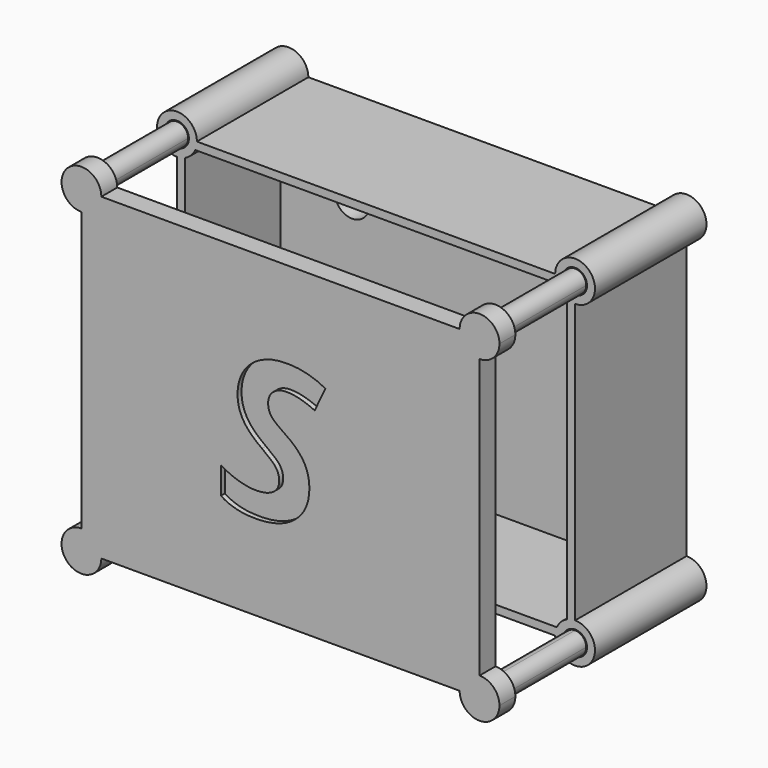
from build123d import *

# Parameters (mm, degrees)
F0_R         = 2.778125
F1_DEPTH     = 3.175
F2_DEPTH     = 22.225
F3_W         = 3.175
F3_H         = 50.8
F4_DEPTH     = 31.75
F6_DEPTH     = 3.175
F7_DEPTH     = 19.05
F5_TEXT_SIZE = 31.9108936108
F8_DEPTH     = 0.79375


# Not quite as in the source:
# - a length typed as a fraction of an inch, garbled in the dataset ("3 / 203.2 mm" for 3/8 in), is restored
# - Text() gives the source's letters only with a copy of the font that has no kerning and outlines rounded to 1/6400 em; it was checked with that copy


with BuildPart() as f1:
    # F0 (on Front) → F1 (new body)
    with BuildSketch(Plane.XZ):
        with BuildLine():
            Line((28.8400644337, 24.13), (-28.8400644337, 24.13))
            ThreePointArc((-28.8400644337, 24.13), (-29.5049359697, 23.1549359697), (-30.48, 22.4900644337))
            Line((-30.48, 22.4900644337), (-30.48, -22.4900644337))
            ThreePointArc((-30.48, -22.4900644337), (-29.5049359697, -23.1549359697), (-28.8400644337, -24.13))
            Line((-28.8400644337, -24.13), (28.8400644337, -24.13))
            ThreePointArc((28.8400644337, -24.13), (29.5049359697, -23.1549359697), (30.48, -22.4900644337))
            Line((30.48, -22.4900644337), (30.48, 22.4900644337))
            ThreePointArc((30.48, 22.4900644337), (29.5049359697, 23.1549359697), (28.8400644337, 24.13))
        make_face()
        with Locations((-19.05, 12.7)):
            Circle(F0_R, mode=Mode.SUBTRACT)
        with BuildLine():
            ThreePointArc((-30.48, 22.4900644337), (-31.1013168813, 22.2919724564), (-31.75, 22.225))
            Line((-31.75, 22.225), (-31.75, -22.225))
            ThreePointArc((-31.75, -22.225), (-31.1013168813, -22.2919724564), (-30.48, -22.4900644337))
            Line((-30.48, -22.4900644337), (-30.48, 22.4900644337))
        make_face()
        with BuildLine():
            ThreePointArc((-28.8400644337, 24.13), (-28.6419724564, 24.7513168813), (-28.575, 25.4))
            Line((-28.575, 25.4), (-29.845, 25.4))
            ThreePointArc((-29.845, 25.4), (-29.9704016562, 24.720253919), (-30.3300968343, 24.13))
            Line((-30.3300968343, 24.13), (-28.8400644337, 24.13))
        make_face()
        with BuildLine():
            Line((-29.845, 25.4), (-28.575, 25.4))
            ThreePointArc((-28.575, 25.4), (-33.9950640303, 27.6450640303), (-31.75, 22.225))
            Line((-31.75, 22.225), (-31.75, 23.495))
            ThreePointArc((-31.75, 23.495), (-33.0970384182, 26.7470384182), (-29.845, 25.4))
        make_face()
        with BuildLine():
            Line((28.575, 25.4), (-28.575, 25.4))
            ThreePointArc((-28.575, 25.4), (-28.6419724564, 24.7513168813), (-28.8400644337, 24.13))
            Line((-28.8400644337, 24.13), (28.8400644337, 24.13))
            ThreePointArc((28.8400644337, 24.13), (28.6419724564, 24.7513168813), (28.575, 25.4))
        make_face()
        with BuildLine():
            ThreePointArc((34.925, 25.4), (31.75, 28.575), (28.575, 25.4))
            Line((28.575, 25.4), (29.845, 25.4))
            ThreePointArc((29.845, 25.4), (31.75, 27.305), (33.655, 25.4))
            ThreePointArc((33.655, 25.4), (33.0970384182, 24.0529615818), (31.75, 23.495))
            Line((31.75, 23.495), (31.75, 22.225))
            ThreePointArc((31.75, 22.225), (33.9950640303, 23.1549359697), (34.925, 25.4))
        make_face()
        with BuildLine():
            Line((29.845, 25.4), (28.575, 25.4))
            ThreePointArc((28.575, 25.4), (28.6419724564, 24.7513168813), (28.8400644337, 24.13))
            Line((28.8400644337, 24.13), (30.3300968343, 24.13))
            ThreePointArc((30.3300968343, 24.13), (29.9704016562, 24.720253919), (29.845, 25.4))
        make_face()
        with BuildLine():
            Line((-31.75, 23.495), (-31.75, 22.225))
            ThreePointArc((-31.75, 22.225), (-31.1013168813, 22.2919724564), (-30.48, 22.4900644337))
            Line((-30.48, 22.4900644337), (-30.48, 23.9800968343))
            ThreePointArc((-30.48, 23.9800968343), (-31.070253919, 23.6204016562), (-31.75, 23.495))
        make_face()
        with BuildLine():
            ThreePointArc((-30.48, -22.4900644337), (-31.1013168813, -22.2919724564), (-31.75, -22.225))
            Line((-31.75, -22.225), (-31.75, -23.4950015545))
            ThreePointArc((-31.75, -23.4950015545), (-31.0702538242, -23.6204033564), (-30.48, -23.9800989199))
            Line((-30.48, -23.9800989199), (-30.48, -22.4900644337))
        make_face()
        with BuildLine():
            Line((-31.75, -23.4950015545), (-31.75, -22.225))
            ThreePointArc((-31.75, -22.225), (-33.9950640303, -27.6450640303), (-28.575, -25.4))
            Line((-28.575, -25.4), (-29.8450015545, -25.4))
            ThreePointArc((-29.8450015545, -25.4), (-33.097037319, -26.747037319), (-31.75, -23.4950015545))
        make_face()
        with BuildLine():
            ThreePointArc((30.48, 22.4900644337), (31.1013168813, 22.2919724564), (31.75, 22.225))
            Line((31.75, 22.225), (31.75, 23.495))
            ThreePointArc((31.75, 23.495), (31.070253919, 23.6204016562), (30.48, 23.9800968343))
            Line((30.48, 23.9800968343), (30.48, 22.4900644337))
        make_face()
        with BuildLine():
            Line((31.75, -22.225), (31.75, 22.225))
            ThreePointArc((31.75, 22.225), (31.1013168813, 22.2919724564), (30.48, 22.4900644337))
            Line((30.48, 22.4900644337), (30.48, -22.4900644337))
            ThreePointArc((30.48, -22.4900644337), (31.1013168813, -22.2919724564), (31.75, -22.225))
        make_face()
        with BuildLine():
            ThreePointArc((-28.8400644337, -24.13), (-28.6419724564, -24.7513168813), (-28.575, -25.4))
            Line((-28.575, -25.4), (28.575, -25.4))
            ThreePointArc((28.575, -25.4), (28.6419724564, -24.7513168813), (28.8400644337, -24.13))
            Line((28.8400644337, -24.13), (-28.8400644337, -24.13))
        make_face()
        with BuildLine():
            Line((-29.8450015545, -25.4), (-28.575, -25.4))
            ThreePointArc((-28.575, -25.4), (-28.6419724564, -24.7513168813), (-28.8400644337, -24.13))
            Line((-28.8400644337, -24.13), (-30.3300989199, -24.13))
            ThreePointArc((-30.3300989199, -24.13), (-29.9704033564, -24.7202538242), (-29.8450015545, -25.4))
        make_face()
        with BuildLine():
            ThreePointArc((34.925, -25.4), (33.9950640303, -23.1549359697), (31.75, -22.225))
            Line((31.75, -22.225), (31.75, -23.495))
            ThreePointArc((31.75, -23.495), (33.0970384182, -24.0529615818), (33.655, -25.4))
            ThreePointArc((33.655, -25.4), (31.75, -27.305), (29.845, -25.4))
            Line((29.845, -25.4), (28.575, -25.4))
            ThreePointArc((28.575, -25.4), (31.75, -28.575), (34.925, -25.4))
        make_face()
        with BuildLine():
            Line((31.75, -23.495), (31.75, -22.225))
            ThreePointArc((31.75, -22.225), (31.1013168813, -22.2919724564), (30.48, -22.4900644337))
            Line((30.48, -22.4900644337), (30.48, -23.9800968343))
            ThreePointArc((30.48, -23.9800968343), (31.070253919, -23.6204016562), (31.75, -23.495))
        make_face()
        with BuildLine():
            ThreePointArc((28.8400644337, -24.13), (28.6419724564, -24.7513168813), (28.575, -25.4))
            Line((28.575, -25.4), (29.845, -25.4))
            ThreePointArc((29.845, -25.4), (29.9704016562, -24.720253919), (30.3300968343, -24.13))
            Line((30.3300968343, -24.13), (28.8400644337, -24.13))
        make_face()
        with BuildLine():
            ThreePointArc((-30.48, 22.4900644337), (-29.5049359697, 23.1549359697), (-28.8400644337, 24.13))
            Line((-28.8400644337, 24.13), (-30.3300968343, 24.13))
            ThreePointArc((-30.3300968343, 24.13), (-30.4029615818, 24.0529615818), (-30.48, 23.9800968343))
            Line((-30.48, 23.9800968343), (-30.48, 22.4900644337))
        make_face()
        with BuildLine():
            ThreePointArc((-28.8400644337, -24.13), (-29.5049359697, -23.1549359697), (-30.48, -22.4900644337))
            Line((-30.48, -22.4900644337), (-30.48, -23.9800989199))
            ThreePointArc((-30.48, -23.9800989199), (-30.402962681, -24.052962681), (-30.3300989199, -24.13))
            Line((-30.3300989199, -24.13), (-28.8400644337, -24.13))
        make_face()
        with BuildLine():
            Line((30.48, -23.9800968343), (30.48, -22.4900644337))
            ThreePointArc((30.48, -22.4900644337), (29.5049359697, -23.1549359697), (28.8400644337, -24.13))
            Line((28.8400644337, -24.13), (30.3300968343, -24.13))
            ThreePointArc((30.3300968343, -24.13), (30.4029615818, -24.0529615818), (30.48, -23.9800968343))
        make_face()
        with BuildLine():
            Line((30.3300968343, 24.13), (28.8400644337, 24.13))
            ThreePointArc((28.8400644337, 24.13), (29.5049359697, 23.1549359697), (30.48, 22.4900644337))
            Line((30.48, 22.4900644337), (30.48, 23.9800968343))
            ThreePointArc((30.48, 23.9800968343), (30.4029615818, 24.0529615818), (30.3300968343, 24.13))
        make_face()
        with BuildLine():
            ThreePointArc((-30.3300968343, 24.13), (-29.9704016562, 24.720253919), (-29.845, 25.4))
            Line((-29.845, 25.4), (-31.75, 25.4))
            Line((-31.75, 25.4), (-31.75, 23.495))
            ThreePointArc((-31.75, 23.495), (-31.070253919, 23.6204016562), (-30.48, 23.9800968343))
            Line((-30.48, 23.9800968343), (-30.48, 24.13))
            Line((-30.48, 24.13), (-30.3300968343, 24.13))
        make_face()
        with BuildLine():
            Line((-31.75, 25.4), (-29.845, 25.4))
            ThreePointArc((-29.845, 25.4), (-33.0970384182, 26.7470384182), (-31.75, 23.495))
            Line((-31.75, 23.495), (-31.75, 25.4))
        make_face()
        with BuildLine():
            ThreePointArc((33.655, 25.4), (31.75, 27.305), (29.845, 25.4))
            Line((29.845, 25.4), (31.75, 25.4))
            Line((31.75, 25.4), (31.75, 23.495))
            ThreePointArc((31.75, 23.495), (33.0970384182, 24.0529615818), (33.655, 25.4))
        make_face()
        with BuildLine():
            Line((31.75, 25.4), (29.845, 25.4))
            ThreePointArc((29.845, 25.4), (29.9704016562, 24.720253919), (30.3300968343, 24.13))
            Line((30.3300968343, 24.13), (30.48, 24.13))
            Line((30.48, 24.13), (30.48, 23.9800968343))
            ThreePointArc((30.48, 23.9800968343), (31.070253919, 23.6204016562), (31.75, 23.495))
            Line((31.75, 23.495), (31.75, 25.4))
        make_face()
        with BuildLine():
            ThreePointArc((33.655, -25.4), (33.0970384182, -24.0529615818), (31.75, -23.495))
            Line((31.75, -23.495), (31.75, -25.4))
            Line((31.75, -25.4), (29.845, -25.4))
            ThreePointArc((29.845, -25.4), (31.75, -27.305), (33.655, -25.4))
        make_face()
        with BuildLine():
            Line((31.75, -25.4), (31.75, -23.495))
            ThreePointArc((31.75, -23.495), (31.070253919, -23.6204016562), (30.48, -23.9800968343))
            Line((30.48, -23.9800968343), (30.48, -24.13))
            Line((30.48, -24.13), (30.3300968343, -24.13))
            ThreePointArc((30.3300968343, -24.13), (29.9704016562, -24.720253919), (29.845, -25.4))
            Line((29.845, -25.4), (31.75, -25.4))
        make_face()
        with BuildLine():
            ThreePointArc((-30.48, -23.9800989199), (-31.0702538242, -23.6204033564), (-31.75, -23.4950015545))
            Line((-31.75, -23.4950015545), (-31.75, -25.4))
            Line((-31.75, -25.4), (-29.8450015545, -25.4))
            ThreePointArc((-29.8450015545, -25.4), (-29.9704033564, -24.7202538242), (-30.3300989199, -24.13))
            Line((-30.3300989199, -24.13), (-30.48, -24.13))
            Line((-30.48, -24.13), (-30.48, -23.9800989199))
        make_face()
        with BuildLine():
            Line((-31.75, -25.4), (-31.75, -23.4950015545))
            ThreePointArc((-31.75, -23.4950015545), (-33.097037319, -26.747037319), (-29.8450015545, -25.4))
            Line((-29.8450015545, -25.4), (-31.75, -25.4))
        make_face()
    extrude(amount=F1_DEPTH)

    # F0 (on Front) → F2 (join)
    with BuildSketch(Plane.XZ):
        with BuildLine():
            ThreePointArc((-30.48, 22.4900644337), (-31.1013168813, 22.2919724564), (-31.75, 22.225))
            Line((-31.75, 22.225), (-31.75, -22.225))
            ThreePointArc((-31.75, -22.225), (-31.1013168813, -22.2919724564), (-30.48, -22.4900644337))
            Line((-30.48, -22.4900644337), (-30.48, 22.4900644337))
        make_face()
        with BuildLine():
            ThreePointArc((-28.8400644337, -24.13), (-28.6419724564, -24.7513168813), (-28.575, -25.4))
            Line((-28.575, -25.4), (28.575, -25.4))
            ThreePointArc((28.575, -25.4), (28.6419724564, -24.7513168813), (28.8400644337, -24.13))
            Line((28.8400644337, -24.13), (-28.8400644337, -24.13))
        make_face()
        with BuildLine():
            Line((31.75, -22.225), (31.75, 22.225))
            ThreePointArc((31.75, 22.225), (31.1013168813, 22.2919724564), (30.48, 22.4900644337))
            Line((30.48, 22.4900644337), (30.48, -22.4900644337))
            ThreePointArc((30.48, -22.4900644337), (31.1013168813, -22.2919724564), (31.75, -22.225))
        make_face()
        with BuildLine():
            Line((28.575, 25.4), (-28.575, 25.4))
            ThreePointArc((-28.575, 25.4), (-28.6419724564, 24.7513168813), (-28.8400644337, 24.13))
            Line((-28.8400644337, 24.13), (28.8400644337, 24.13))
            ThreePointArc((28.8400644337, 24.13), (28.6419724564, 24.7513168813), (28.575, 25.4))
        make_face()
        with BuildLine():
            Line((30.3300968343, 24.13), (28.8400644337, 24.13))
            ThreePointArc((28.8400644337, 24.13), (29.5049359697, 23.1549359697), (30.48, 22.4900644337))
            Line((30.48, 22.4900644337), (30.48, 23.9800968343))
            ThreePointArc((30.48, 23.9800968343), (30.4029615818, 24.0529615818), (30.3300968343, 24.13))
        make_face()
        with BuildLine():
            ThreePointArc((30.48, 22.4900644337), (31.1013168813, 22.2919724564), (31.75, 22.225))
            Line((31.75, 22.225), (31.75, 23.495))
            ThreePointArc((31.75, 23.495), (31.070253919, 23.6204016562), (30.48, 23.9800968343))
            Line((30.48, 23.9800968343), (30.48, 22.4900644337))
        make_face()
        with BuildLine():
            Line((29.845, 25.4), (28.575, 25.4))
            ThreePointArc((28.575, 25.4), (28.6419724564, 24.7513168813), (28.8400644337, 24.13))
            Line((28.8400644337, 24.13), (30.3300968343, 24.13))
            ThreePointArc((30.3300968343, 24.13), (29.9704016562, 24.720253919), (29.845, 25.4))
        make_face()
        with BuildLine():
            ThreePointArc((34.925, 25.4), (31.75, 28.575), (28.575, 25.4))
            Line((28.575, 25.4), (29.845, 25.4))
            ThreePointArc((29.845, 25.4), (31.75, 27.305), (33.655, 25.4))
            ThreePointArc((33.655, 25.4), (33.0970384182, 24.0529615818), (31.75, 23.495))
            Line((31.75, 23.495), (31.75, 22.225))
            ThreePointArc((31.75, 22.225), (33.9950640303, 23.1549359697), (34.925, 25.4))
        make_face()
        with BuildLine():
            Line((30.48, -23.9800968343), (30.48, -22.4900644337))
            ThreePointArc((30.48, -22.4900644337), (29.5049359697, -23.1549359697), (28.8400644337, -24.13))
            Line((28.8400644337, -24.13), (30.3300968343, -24.13))
            ThreePointArc((30.3300968343, -24.13), (30.4029615818, -24.0529615818), (30.48, -23.9800968343))
        make_face()
        with BuildLine():
            ThreePointArc((28.8400644337, -24.13), (28.6419724564, -24.7513168813), (28.575, -25.4))
            Line((28.575, -25.4), (29.845, -25.4))
            ThreePointArc((29.845, -25.4), (29.9704016562, -24.720253919), (30.3300968343, -24.13))
            Line((30.3300968343, -24.13), (28.8400644337, -24.13))
        make_face()
        with BuildLine():
            Line((31.75, -23.495), (31.75, -22.225))
            ThreePointArc((31.75, -22.225), (31.1013168813, -22.2919724564), (30.48, -22.4900644337))
            Line((30.48, -22.4900644337), (30.48, -23.9800968343))
            ThreePointArc((30.48, -23.9800968343), (31.070253919, -23.6204016562), (31.75, -23.495))
        make_face()
        with BuildLine():
            ThreePointArc((34.925, -25.4), (33.9950640303, -23.1549359697), (31.75, -22.225))
            Line((31.75, -22.225), (31.75, -23.495))
            ThreePointArc((31.75, -23.495), (33.0970384182, -24.0529615818), (33.655, -25.4))
            ThreePointArc((33.655, -25.4), (31.75, -27.305), (29.845, -25.4))
            Line((29.845, -25.4), (28.575, -25.4))
            ThreePointArc((28.575, -25.4), (31.75, -28.575), (34.925, -25.4))
        make_face()
        with BuildLine():
            Line((-31.75, -23.4950015545), (-31.75, -22.225))
            ThreePointArc((-31.75, -22.225), (-33.9950640303, -27.6450640303), (-28.575, -25.4))
            Line((-28.575, -25.4), (-29.8450015545, -25.4))
            ThreePointArc((-29.8450015545, -25.4), (-33.097037319, -26.747037319), (-31.75, -23.4950015545))
        make_face()
        with BuildLine():
            ThreePointArc((-30.48, -22.4900644337), (-31.1013168813, -22.2919724564), (-31.75, -22.225))
            Line((-31.75, -22.225), (-31.75, -23.4950015545))
            ThreePointArc((-31.75, -23.4950015545), (-31.0702538242, -23.6204033564), (-30.48, -23.9800989199))
            Line((-30.48, -23.9800989199), (-30.48, -22.4900644337))
        make_face()
        with BuildLine():
            ThreePointArc((-28.8400644337, -24.13), (-29.5049359697, -23.1549359697), (-30.48, -22.4900644337))
            Line((-30.48, -22.4900644337), (-30.48, -23.9800989199))
            ThreePointArc((-30.48, -23.9800989199), (-30.402962681, -24.052962681), (-30.3300989199, -24.13))
            Line((-30.3300989199, -24.13), (-28.8400644337, -24.13))
        make_face()
        with BuildLine():
            Line((-29.8450015545, -25.4), (-28.575, -25.4))
            ThreePointArc((-28.575, -25.4), (-28.6419724564, -24.7513168813), (-28.8400644337, -24.13))
            Line((-28.8400644337, -24.13), (-30.3300989199, -24.13))
            ThreePointArc((-30.3300989199, -24.13), (-29.9704033564, -24.7202538242), (-29.8450015545, -25.4))
        make_face()
        with BuildLine():
            ThreePointArc((-28.8400644337, 24.13), (-28.6419724564, 24.7513168813), (-28.575, 25.4))
            Line((-28.575, 25.4), (-29.845, 25.4))
            ThreePointArc((-29.845, 25.4), (-29.9704016562, 24.720253919), (-30.3300968343, 24.13))
            Line((-30.3300968343, 24.13), (-28.8400644337, 24.13))
        make_face()
        with BuildLine():
            ThreePointArc((-30.48, 22.4900644337), (-29.5049359697, 23.1549359697), (-28.8400644337, 24.13))
            Line((-28.8400644337, 24.13), (-30.3300968343, 24.13))
            ThreePointArc((-30.3300968343, 24.13), (-30.4029615818, 24.0529615818), (-30.48, 23.9800968343))
            Line((-30.48, 23.9800968343), (-30.48, 22.4900644337))
        make_face()
        with BuildLine():
            Line((-31.75, 23.495), (-31.75, 22.225))
            ThreePointArc((-31.75, 22.225), (-31.1013168813, 22.2919724564), (-30.48, 22.4900644337))
            Line((-30.48, 22.4900644337), (-30.48, 23.9800968343))
            ThreePointArc((-30.48, 23.9800968343), (-31.070253919, 23.6204016562), (-31.75, 23.495))
        make_face()
        with BuildLine():
            Line((-29.845, 25.4), (-28.575, 25.4))
            ThreePointArc((-28.575, 25.4), (-33.9950640303, 27.6450640303), (-31.75, 22.225))
            Line((-31.75, 22.225), (-31.75, 23.495))
            ThreePointArc((-31.75, 23.495), (-33.0970384182, 26.7470384182), (-29.845, 25.4))
        make_face()
    extrude(amount=F2_DEPTH)


with BuildPart() as f4:
    # F3 (on Right) → F4 (new body, symmetric)
    with BuildSketch(Plane.YZ):
        with Locations((-39.6875, 0)):
            Rectangle(F3_W, F3_H)
    extrude(amount=F4_DEPTH, both=True)

    # F5 (on face) → F6 (join)
    with BuildSketch(Plane.XZ.offset(41.275)):
        with BuildLine():
            ThreePointArc((34.925, 25.4), (31.75, 28.575), (28.575, 25.4))
            Line((28.575, 25.4), (29.972, 25.4))
            ThreePointArc((29.972, 25.4), (31.75, 27.178), (33.528, 25.4))
            ThreePointArc((33.528, 25.4), (33.0072358569, 24.1427641431), (31.75, 23.622))
            Line((31.75, 23.622), (31.75, 22.225))
            ThreePointArc((31.75, 22.225), (33.9950640303, 23.1549359697), (34.925, 25.4))
        make_face()
        with BuildLine():
            ThreePointArc((33.528, 25.4), (31.75, 27.178), (29.972, 25.4))
            Line((29.972, 25.4), (31.75, 25.4))
            Line((31.75, 25.4), (31.75, 23.622))
            ThreePointArc((31.75, 23.622), (33.0072358569, 24.1427641431), (33.528, 25.4))
        make_face()
        with BuildLine():
            ThreePointArc((34.925, -25.4), (33.9950640303, -23.1549359697), (31.75, -22.225))
            Line((31.75, -22.225), (31.75, -23.622))
            ThreePointArc((31.75, -23.622), (33.0072358569, -24.1427641431), (33.528, -25.4))
            ThreePointArc((33.528, -25.4), (31.75, -27.178), (29.972, -25.4))
            Line((29.972, -25.4), (28.575, -25.4))
            ThreePointArc((28.575, -25.4), (31.75, -28.575), (34.925, -25.4))
        make_face()
        with BuildLine():
            ThreePointArc((33.528, -25.4), (33.0072358569, -24.1427641431), (31.75, -23.622))
            Line((31.75, -23.622), (31.75, -25.4))
            Line((31.75, -25.4), (29.972, -25.4))
            ThreePointArc((29.972, -25.4), (31.75, -27.178), (33.528, -25.4))
        make_face()
        with BuildLine():
            Line((-31.75, -23.622), (-31.75, -22.225))
            ThreePointArc((-31.75, -22.225), (-33.9950640303, -27.6450640303), (-28.575, -25.4))
            Line((-28.575, -25.4), (-29.972, -25.4))
            ThreePointArc((-29.972, -25.4), (-33.0072358569, -26.6572358569), (-31.75, -23.622))
        make_face()
        with BuildLine():
            Line((-31.75, -25.4), (-31.75, -23.622))
            ThreePointArc((-31.75, -23.622), (-33.0072358569, -26.6572358569), (-29.972, -25.4))
            Line((-29.972, -25.4), (-31.75, -25.4))
        make_face()
        with BuildLine():
            ThreePointArc((-29.972, -25.4), (-30.4927641431, -24.1427641431), (-31.75, -23.622))
            Line((-31.75, -23.622), (-31.75, -25.4))
            Line((-31.75, -25.4), (-29.972, -25.4))
        make_face()
        with BuildLine():
            ThreePointArc((-28.575, -25.4), (-29.5049359697, -23.1549359697), (-31.75, -22.225))
            Line((-31.75, -22.225), (-31.75, -23.622))
            ThreePointArc((-31.75, -23.622), (-30.4927641431, -24.1427641431), (-29.972, -25.4))
            Line((-29.972, -25.4), (-28.575, -25.4))
        make_face()
        with BuildLine():
            Line((31.75, -23.622), (31.75, -22.225))
            ThreePointArc((31.75, -22.225), (29.5049359697, -23.1549359697), (28.575, -25.4))
            Line((28.575, -25.4), (29.972, -25.4))
            ThreePointArc((29.972, -25.4), (30.4927641431, -24.1427641431), (31.75, -23.622))
        make_face()
        with BuildLine():
            Line((31.75, -25.4), (31.75, -23.622))
            ThreePointArc((31.75, -23.622), (30.4927641431, -24.1427641431), (29.972, -25.4))
            Line((29.972, -25.4), (31.75, -25.4))
        make_face()
        with BuildLine():
            Line((29.972, 25.4), (28.575, 25.4))
            ThreePointArc((28.575, 25.4), (29.5049359697, 23.1549359697), (31.75, 22.225))
            Line((31.75, 22.225), (31.75, 23.622))
            ThreePointArc((31.75, 23.622), (30.4927641431, 24.1427641431), (29.972, 25.4))
        make_face()
        with BuildLine():
            Line((31.75, 25.4), (29.972, 25.4))
            ThreePointArc((29.972, 25.4), (30.4927641431, 24.1427641431), (31.75, 23.622))
            Line((31.75, 23.622), (31.75, 25.4))
        make_face()
        with BuildLine():
            ThreePointArc((-31.75, 23.622), (-30.4927641431, 24.1427641431), (-29.972, 25.4))
            Line((-29.972, 25.4), (-31.75, 25.4))
            Line((-31.75, 25.4), (-31.75, 23.622))
        make_face()
        with BuildLine():
            ThreePointArc((-31.75, 22.225), (-29.5049359697, 23.1549359697), (-28.575, 25.4))
            Line((-28.575, 25.4), (-29.972, 25.4))
            ThreePointArc((-29.972, 25.4), (-30.4927641431, 24.1427641431), (-31.75, 23.622))
            Line((-31.75, 23.622), (-31.75, 22.225))
        make_face()
        with BuildLine():
            Line((-31.75, 25.4), (-29.972, 25.4))
            ThreePointArc((-29.972, 25.4), (-33.0072358569, 26.6572358569), (-31.75, 23.622))
            Line((-31.75, 23.622), (-31.75, 25.4))
        make_face()
        with BuildLine():
            Line((-29.972, 25.4), (-28.575, 25.4))
            ThreePointArc((-28.575, 25.4), (-33.9950640303, 27.6450640303), (-31.75, 22.225))
            Line((-31.75, 22.225), (-31.75, 23.622))
            ThreePointArc((-31.75, 23.622), (-33.0072358569, 26.6572358569), (-29.972, 25.4))
        make_face()
    extrude(amount=-F6_DEPTH)

    # F5 (on face) → F7 (join)
    with BuildSketch(Plane.XZ.offset(41.275)):
        with BuildLine():
            Line((-31.75, 25.4), (-29.972, 25.4))
            ThreePointArc((-29.972, 25.4), (-33.0072358569, 26.6572358569), (-31.75, 23.622))
            Line((-31.75, 23.622), (-31.75, 25.4))
        make_face()
        with BuildLine():
            ThreePointArc((-31.75, 23.622), (-30.4927641431, 24.1427641431), (-29.972, 25.4))
            Line((-29.972, 25.4), (-31.75, 25.4))
            Line((-31.75, 25.4), (-31.75, 23.622))
        make_face()
        with BuildLine():
            ThreePointArc((33.528, 25.4), (31.75, 27.178), (29.972, 25.4))
            Line((29.972, 25.4), (31.75, 25.4))
            Line((31.75, 25.4), (31.75, 23.622))
            ThreePointArc((31.75, 23.622), (33.0072358569, 24.1427641431), (33.528, 25.4))
        make_face()
        with BuildLine():
            Line((31.75, 25.4), (29.972, 25.4))
            ThreePointArc((29.972, 25.4), (30.4927641431, 24.1427641431), (31.75, 23.622))
            Line((31.75, 23.622), (31.75, 25.4))
        make_face()
        with BuildLine():
            ThreePointArc((33.528, -25.4), (33.0072358569, -24.1427641431), (31.75, -23.622))
            Line((31.75, -23.622), (31.75, -25.4))
            Line((31.75, -25.4), (29.972, -25.4))
            ThreePointArc((29.972, -25.4), (31.75, -27.178), (33.528, -25.4))
        make_face()
        with BuildLine():
            Line((31.75, -25.4), (31.75, -23.622))
            ThreePointArc((31.75, -23.622), (30.4927641431, -24.1427641431), (29.972, -25.4))
            Line((29.972, -25.4), (31.75, -25.4))
        make_face()
        with BuildLine():
            Line((-31.75, -25.4), (-31.75, -23.622))
            ThreePointArc((-31.75, -23.622), (-33.0072358569, -26.6572358569), (-29.972, -25.4))
            Line((-29.972, -25.4), (-31.75, -25.4))
        make_face()
        with BuildLine():
            ThreePointArc((-29.972, -25.4), (-30.4927641431, -24.1427641431), (-31.75, -23.622))
            Line((-31.75, -23.622), (-31.75, -25.4))
            Line((-31.75, -25.4), (-29.972, -25.4))
        make_face()
    extrude(amount=-F7_DEPTH)

    # F5 (on face) → F8 (cut)
    with BuildSketch(Plane.XZ.offset(41.275)):
        with Locations((-10.1364022121, -11.4879216999)):
            Text('S', F5_TEXT_SIZE, font='Open Sans', font_style=FontStyle.BOLDITALIC, text_align=(TextAlign.LEFT, TextAlign.BOTTOM))
    extrude(amount=-F8_DEPTH, mode=Mode.SUBTRACT)


solid = Compound([f1.part, f4.part])
